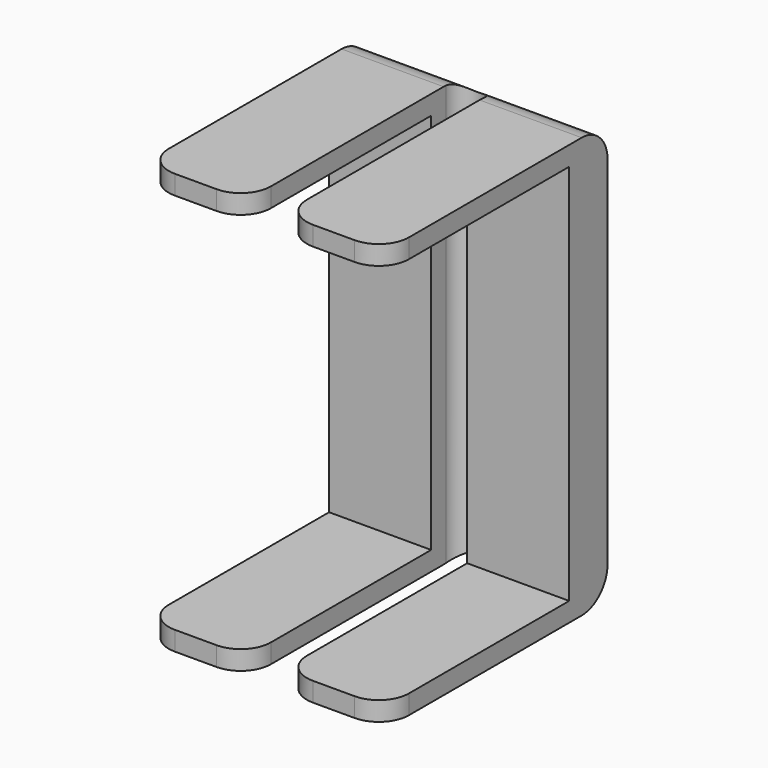
from build123d import *

# Parameters (mm, degrees)
F1_DEPTH    = 25
F2_DEPTH    = 1
F4_DEPTH    = 47.5
F5_R        = 3.1384776311
F6_T1_DEPTH = 41.8994949366


# Not quite as in the source:
# - a fillet or chamfer that OpenCascade refuses, or shapes differently, is made with other operations: its cross-section is extruded or revolved along the edge and cut away or added


with BuildPart() as f1:
    # F0 (on Right) → F1 (new body)
    with BuildSketch(Plane.YZ):
        Polygon((0, 43.8), (-29, 43.8), (-29, 41.8), (-4, 41.8), (-4, 2), (-29, 2), (-29, 0), (0, 0), align=None)
    extrude(amount=F1_DEPTH)

    # F2 (add): a face of the model
    f2_faces = [f1.faces().sort_by_distance(p)[0] for p in [
        (12.5, -4, 21.9),
    ]]
    extrude(f2_faces, amount=F2_DEPTH)

    # F3 (on face) → F4 (cut)
    with BuildSketch(Plane.XY.offset(43.8)):
        with BuildLine():
            Line((12.5, -3.075), (14.375, -3.075))
            ThreePointArc((14.375, -3.075), (12.5, -1.2), (10.625, -3.075))
            Line((10.625, -3.075), (12.5, -3.075))
        make_face()
        with BuildLine():
            Line((14.375, -29), (14.375, -3.075))
            ThreePointArc((14.375, -3.075), (12.5, -4.95), (10.625, -3.075))
            Line((10.625, -3.075), (10.625, -29))
            Line((10.625, -29), (14.375, -29))
        make_face()
        with BuildLine():
            ThreePointArc((10.625, -3.075), (12.5, -4.95), (14.375, -3.075))
            Line((14.375, -3.075), (12.5, -3.075))
            Line((12.5, -3.075), (10.625, -3.075))
        make_face()
    extrude(amount=-F4_DEPTH, mode=Mode.SUBTRACT)

    # F5
    f5_edges = [f1.edges().sort_by_distance(p)[0] for p in [
        (0, -29, 42.8),
        (10.625, -29, 42.8),
        (14.375, -29, 42.8),
        (25, -29, 42.8),
        (25, -29, 1),
        (14.375, -29, 1),
        (10.625, -29, 1),
        (0, -29, 1),
    ]]
    fillet(f5_edges, radius=F5_R)

    # F6: fillet of radius 3.3798989873 on 2 edges, made by hand

    # F6_s2 → F6_t1 (cut)
    with BuildSketch(Plane.YZ.offset(-8.4497474683)):
        with BuildLine():
            ThreePointArc((-3.3798989873, 43.8), (-0.9899494937, 42.8100505063), (0, 40.4201010127))
            Line((0, 40.4201010127), (0, 43.8))
            Line((0, 43.8), (-3.3798989873, 43.8))
        make_face()
        with BuildLine():
            ThreePointArc((0, 3.3798989873), (-0.9899494937, 0.9899494937), (-3.3798989873, 0))
            Line((-3.3798989873, 0), (0, 0))
            Line((0, 0), (0, 3.3798989873))
        make_face()
    extrude(amount=F6_T1_DEPTH, mode=Mode.SUBTRACT)


solid = f1.part
